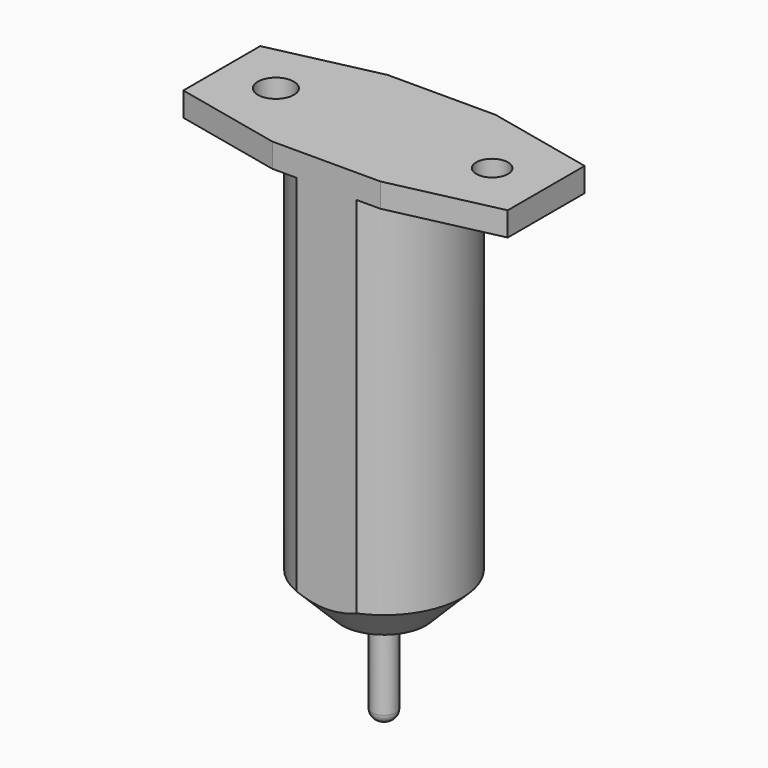
from build123d import *

# Parameters (mm, degrees)
F0_R      = 6.5
F1_DEPTH  = 33.3
F2_SIZE   = 3
F3_W      = 27
F3_H      = 12
F4_DEPTH  = 2
F5_R      = 1
F6_DEPTH  = 8
F7_R      = 0.8
F8_R      = 1.5
F8_R_2    = 1.3212801888
F9_DEPTH  = 25
F11_DEPTH = 2
F12_W     = 9
F12_H     = 44.6074357137
F13_DEPTH = 5
F14_W     = 9
F14_H     = 35.2907052629
F15_DEPTH = 5


with BuildPart() as f1:
    # F0 (on Top) → F1 (new body)
    with BuildSketch(Plane.XY):
        Circle(F0_R)
    extrude(amount=F1_DEPTH)

    # F2
    f2_edges = [f1.edges().sort_by_distance(p)[0] for p in [
        (-6.5, 0, 0),
    ]]
    chamfer(f2_edges, length=F2_SIZE)

    # F3 (on face) → F4 (join)
    with BuildSketch(Plane.XY.offset(33.3)):
        Rectangle(F3_W, F3_H)
    extrude(amount=F4_DEPTH)

    # F5 (on face) → F6 (join)
    with BuildSketch(Plane(origin=(0, 0, 0), x_dir=(1, 0, 0), z_dir=(0, 0, -1))):
        Circle(F5_R)
    extrude(amount=F6_DEPTH)

    # F7
    f7_edges = [f1.edges().sort_by_distance(p)[0] for p in [
        (-1, 0, -8),
    ]]
    fillet(f7_edges, radius=F7_R)

    # F8 (on face) → F9 (cut)
    with BuildSketch(Plane.XY.offset(35.3)):
        with Locations((-9, 0)):
            Circle(F8_R)
        with Locations((9, 0)):
            Circle(F8_R_2)
    extrude(amount=-F9_DEPTH, mode=Mode.SUBTRACT)

    # F10 (on face) → F11 (cut, through all)
    with BuildSketch(Plane.XY.offset(35.3)):
        Polygon((-13.5, -4), (-13.5, -6), (-4.5, -6), align=None)
        Polygon((-4.5, 6), (-13.5, 6), (-13.5, 4), align=None)
        Polygon((13.5, -4), (4.5, -6), (13.5, -6), align=None)
        Polygon((13.5, 4), (13.5, 6), (4.5, 6), align=None)
    extrude(amount=-F11_DEPTH, mode=Mode.SUBTRACT)

    # F12 (on face) → F13 (cut)
    with BuildSketch(Plane.XZ.offset(6)):
        with Locations((0, 12.9962821431)):
            Rectangle(F12_W, F12_H)
    extrude(amount=F13_DEPTH, mode=Mode.SUBTRACT)

    # F14 (on face) → F15 (cut)
    with BuildSketch(Plane(origin=(0, 6, 0), x_dir=(-1, 0, 0), z_dir=(0, 1, 0))):
        with Locations((0, 15.6546473686)):
            Rectangle(F14_W, F14_H)
    extrude(amount=F15_DEPTH, mode=Mode.SUBTRACT)


solid = f1.part
